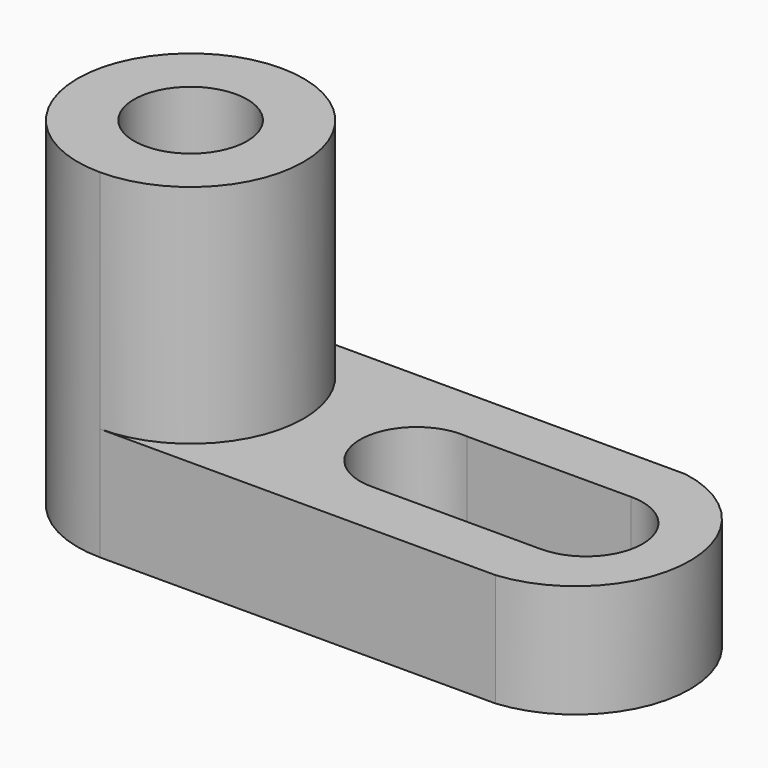
from build123d import *

# Parameters (mm, degrees)
F0_W      = 69.85
F0_H      = 38.1
F1_DEPTH  = 25.4
F5_DEPTH  = 50.8
F7_DEPTH  = 25.4
F8_R      = 6.35
F9_DEPTH  = 50.8
F11_DEPTH = 25.4
F13_DEPTH = 25.4


# Not quite as in the source:
# - a feature of the source that left no trace in its solid (it failed there, or was rolled back) is left out


with BuildPart() as f1:
    # F0 (on Front) → F1 (new body)
    with BuildSketch(Plane.XZ):
        with Locations((34.925, 19.05)):
            Rectangle(F0_W, F0_H)
    extrude(amount=F1_DEPTH)

    # F4 (on face) → F5 (cut)
    with BuildSketch(Plane.XY.offset(38.1)):
        with BuildLine():
            ThreePointArc((0, -12.7), (3.7197438789, -3.7197438789), (12.7, 0))
            Line((12.7, 0), (0, 0))
            Line((0, 0), (0, -12.7))
        make_face()
        with BuildLine():
            Line((0, -25.4), (12.7, -25.4))
            ThreePointArc((12.7, -25.4), (3.7197438789, -21.6802561211), (0, -12.7))
            Line((0, -12.7), (0, -25.4))
        make_face()
    extrude(amount=-F5_DEPTH, mode=Mode.SUBTRACT)

    # F6 (on face) → F7 (cut)
    with BuildSketch(Plane.XY.offset(38.1)):
        with BuildLine():
            ThreePointArc((12.7, 0), (25.4, -12.7), (12.7, -25.4))
            Line((12.7, -25.4), (69.85, -25.4))
            Line((69.85, -25.4), (69.85, 0))
            Line((69.85, 0), (12.7, 0))
        make_face()
    extrude(amount=-F7_DEPTH, mode=Mode.SUBTRACT)

    # F8 (on face) → F9 (cut)
    with BuildSketch(Plane.XY.offset(38.1)):
        with Locations((12.7, -12.7)):
            Circle(F8_R)
    extrude(amount=-F9_DEPTH, mode=Mode.SUBTRACT)

    # F10 (on face) → F11 (cut)
    with BuildSketch(Plane.XY.offset(12.7)):
        with BuildLine():
            ThreePointArc((38.1, -19.05), (42.5901280605, -17.1901280605), (44.45, -12.7))
            ThreePointArc((44.45, -12.7), (42.7995135722, -8.4295114817), (38.7060402567, -6.37898622))
            Line((38.7060402567, -6.37898622), (38.1, -19.05))
        make_face()
        with BuildLine():
            ThreePointArc((38.7060402567, -6.37898622), (42.7995135722, -8.4295114817), (44.45, -12.7))
            ThreePointArc((44.45, -12.7), (42.5901280605, -17.1901280605), (38.1, -19.05))
            Line((38.1, -19.05), (57.15, -19.05))
            ThreePointArc((57.15, -19.05), (50.8000019615, -12.7049911232), (57.1400177568, -6.3500078461))
            Line((57.1400177568, -6.3500078461), (38.7060402567, -6.37898622))
        make_face()
        with BuildLine():
            Line((38.1, -19.05), (38.7060402567, -6.37898622))
            ThreePointArc((38.7060402567, -6.37898622), (31.7572506946, -12.3966334751), (38.1, -19.05))
        make_face()
        with BuildLine():
            Line((57.15, -19.05), (57.1400177568, -6.3500078461))
            ThreePointArc((57.1400177568, -6.3500078461), (50.8000019615, -12.7049911232), (57.15, -19.05))
        make_face()
        with BuildLine():
            ThreePointArc((63.5, -12.7), (61.6365974165, -8.2063440694), (57.1400177568, -6.3500078461))
            Line((57.1400177568, -6.3500078461), (57.15, -19.05))
            ThreePointArc((57.15, -19.05), (61.6401280605, -17.1901280605), (63.5, -12.7))
        make_face()
    extrude(amount=-F11_DEPTH, mode=Mode.SUBTRACT)

    # F12 (on face) → F13 (cut)
    with BuildSketch(Plane.XY.offset(12.7)):
        with BuildLine():
            ThreePointArc((58.1890903413, 0), (68.7523295615, -13.1579480832), (57.1400177568, -25.4))
            Line((57.1400177568, -25.4), (69.85, -25.4))
            Line((69.85, -25.4), (69.85, 0))
            Line((69.85, 0), (58.1890903413, 0))
        make_face()
    extrude(amount=-F13_DEPTH, mode=Mode.SUBTRACT)


solid = f1.part
